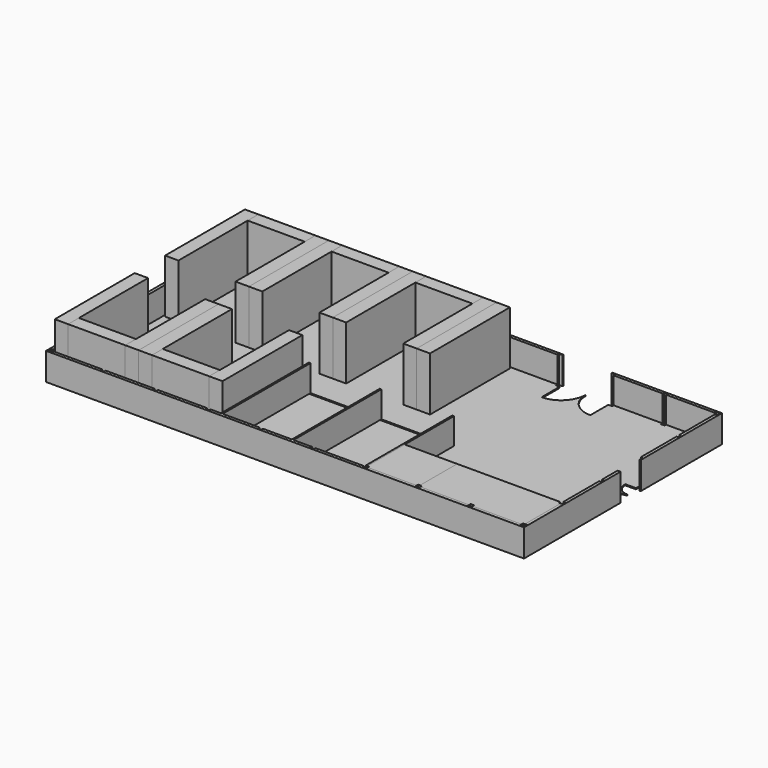
from build123d import *

# Parameters (mm, degrees)
F0_W     = 4500
F0_H     = 1300
F1_DEPTH = 100
F2_DEPTH = 5000
F3_DEPTH = 5000
F4_DEPTH = 5000
F0_W_2   = 150
F0_H_2   = 9850
F0_H_3   = 150
F5_DEPTH = 2500
F6_DEPTH = 2500
F7_DEPTH = 2500
F8_DEPTH = 2500


# Not quite as in the source:
# - a feature names something its author has since deleted; it is built from what else it names


with BuildPart() as f1:
    # F0 (on Top) → F1 (new body)
    with BuildSketch(Plane.XY):
        with BuildLine():
            ThreePointArc((33274.4446, 19781.1111), (31705.4532121104, 20431.0086121104), (31055.5557, 22000))
            ThreePointArc((31055.5557, 22000), (30405.6581878896, 20431.0086121104), (28836.6668, 19781.1111))
            Line((28836.6668, 19781.1111), (28836.6668, 21830))
            Line((28836.6668, 21830), (28496.6668, 21830))
            Line((28496.6668, 21830), (28496.6668, 22000))
            Line((28496.6668, 22000), (24058.889, 22000))
            Line((24058.889, 22000), (24058.889, 21830))
            Line((24058.889, 21830), (24310, 21830))
            Line((24310, 21830), (24310, 12730))
            Line((24310, 12730), (23090, 12730))
            Line((23090, 12730), (21870, 12730))
            Line((21870, 12730), (21870, 20610))
            Line((21870, 20610), (16670, 20610))
            Line((16670, 20610), (16670, 12730))
            Line((16670, 12730), (15450, 12730))
            Line((15450, 12730), (14230, 12730))
            Line((14230, 12730), (14230, 20610))
            Line((14230, 20610), (9030, 20610))
            Line((9030, 20610), (9030, 12730))
            Line((9030, 12730), (7810, 12730))
            Line((7810, 12730), (6590, 12730))
            Line((6590, 12730), (6590, 20610))
            Line((6590, 20610), (1390, 20610))
            Line((1390, 20610), (1390, 12730))
            Line((1390, 12730), (170, 12730))
            Line((170, 12730), (170, 13030))
            Line((170, 13030), (0, 13030))
            Line((0, 13030), (0, 12000))
            Line((0, 12000), (0, 10000))
            Line((0, 10000), (15450, 10000))
            Line((15450, 10000), (15600, 10000))
            Line((15600, 10000), (21908.3334, 10000))
            Line((21908.3334, 10000), (22058.3334, 10000))
            Line((22058.3334, 10000), (28516.6668, 10000))
            Line((28516.6668, 10000), (28666.6668, 10000))
            Line((28666.6668, 10000), (28666.6668, 4400))
            Line((28666.6668, 4400), (33444.4446, 4400))
            Line((33444.4446, 4400), (42830, 4400))
            Line((42830, 4400), (42830, 4570))
            Line((42830, 4570), (43000, 4570))
            Line((43000, 4570), (43000, 8630))
            Line((43000, 8630), (42830, 8630))
            Line((42830, 8630), (42830, 8970))
            Line((42830, 8970), (43000, 8970))
            Line((43000, 8970), (43000, 10730))
            Line((43000, 10730), (41850, 10730))
            ThreePointArc((41850, 10730), (42186.8272016355, 11543.1727983645), (43000, 11880))
            ThreePointArc((43000, 11880), (42186.8272016355, 12216.8272016355), (41850, 13030))
            Line((41850, 13030), (42830, 13030))
            Line((42830, 13030), (42830, 13370))
            Line((42830, 13370), (43000, 13370))
            Line((43000, 13370), (43000, 17430))
            Line((43000, 17430), (42830, 17430))
            Line((42830, 17430), (42830, 17770))
            Line((42830, 17770), (43000, 17770))
            Line((43000, 17770), (43000, 21830))
            Line((43000, 21830), (42830.0002, 21830))
            Line((42830.0002, 21830), (42830.0002, 22000))
            Line((42830.0002, 22000), (38392.2224, 22000))
            Line((38392.2224, 22000), (38392.2224, 21830))
            Line((38392.2224, 21830), (38052.2224, 21830))
            Line((38052.2224, 21830), (38052.2224, 22000))
            Line((38052.2224, 22000), (33614.4446, 22000))
            Line((33614.4446, 22000), (33614.4446, 21830))
            Line((33614.4446, 21830), (33274.4446, 21830))
            Line((33274.4446, 21830), (33274.4446, 19781.1111))
        make_face()
        with Locations((3865.0875091553, 17252.7908325195)):
            Rectangle(F0_W, F0_H, mode=Mode.SUBTRACT)
        with Locations((3865.0875091553, 17252.7908325195)):
            Rectangle(F0_W, F0_H)
        Polygon((15450, 10000), (0, 10000), (0, 8970), (170, 8970), (170, 9270), (1390, 9270), (1390, 1390), (6590, 1390), (6590, 9270), (7810, 9270), (9030, 9270), (9030, 1390), (14230, 1390), (14230, 9270), (15450, 9270), align=None)
        Polygon((33444.4446, 170), (33444.4446, 4400), (28666.6668, 4400), (28666.6668, 170), (28836.6668, 170), (28836.6668, 0), (33274.4446, 0), (33274.4446, 170), align=None)
        Polygon((43000.0001922727, 170), (43000.0000077273, 4230), (42830, 4230), (42830, 4400), (33444.4446, 4400), (33444.4446, 170), (33614.4446, 170), (33614.4446, 0), (38052.2224, 0), (38052.2224, 170), (38392.2224, 170), (38392.2224, 0), (42830.0002, 0), (42830.0002, 170), align=None)
    extrude(amount=F1_DEPTH)

    # F0 (on Top) → F5 (join)
    with BuildSketch(Plane.XY):
        Polygon((15600, 9850), (15600, 10000), (15450, 10000), (15450, 9270), (15450, 170), (15450, 0), (15600, 0), align=None)
        with Locations((21983.3334, 4925)):
            Rectangle(F0_W_2, F0_H_2)
        with Locations((21983.3334, 9925)):
            Rectangle(F0_W_2, F0_H_3)
        Polygon((28666.6668, 170), (28666.6668, 4400), (28666.6668, 10000), (28516.6668, 10000), (28516.6668, 9850), (28516.6668, 4400), (28516.6668, 170), align=None)
    extrude(amount=F5_DEPTH)

    # F0 (on Top) → F6 (join)
    with BuildSketch(Plane.XY):
        Polygon((24058.889, 22000), (28496.6668, 22000), (28496.6668, 22170), (28836.6668, 22170), (28836.6668, 22270), (-270, 22270), (-270, -270), (43270.0002, -270), (43270.0002, 10730), (43000, 10730), (43000, 8970), (43170, 8970), (43170, 8630), (43000, 8630), (43000, 4570), (43170, 4570), (43170, 4230), (43000.0000077273, 4230), (43000.0001922727, 170), (43170.0002, 170), (43170.0002, -170), (42830.0002, -170), (42830.0002, 0), (38392.2224, 0), (38392.2224, -170), (38052.2224, -170), (38052.2224, 0), (33614.4446, 0), (33614.4446, -170), (33274.4446, -170), (33274.4446, 0), (28836.6668, 0), (28836.6668, -170), (28496.6668, -170), (28496.6668, 0), (24058.889, 0), (24058.889, -170), (23718.889, -170), (23718.889, 0), (22058.3334, 0), (21908.3334, 0), (19281.1112, 0), (19281.1112, -170), (18941.1112, -170), (18941.1112, 0), (15600, 0), (15450, 0), (14503.3334, 0), (14503.3334, -170), (14163.3334, -170), (14163.3334, 0), (9725.5556, 0), (9725.5556, -170), (9385.5556, -170), (9385.5556, 0), (4947.7778, 0), (4947.7778, -170), (4607.7778, -170), (4607.7778, 0), (170, 0), (170, -170), (-170, -170), (-170, 170), (0, 170), (0, 4230), (-170, 4230), (-170, 4570), (0, 4570), (0, 8630), (-170, 8630), (-170, 8970), (0, 8970), (0, 10000), (0, 12000), (0, 13030), (-170, 13030), (-170, 13370), (0, 13370), (0, 17430), (-170, 17430), (-170, 17770), (0, 17770), (0, 21830), (-170, 21830), (-170, 22170), (170, 22170), (170, 22000), (4607.7778, 22000), (4607.7778, 22170), (4947.7778, 22170), (4947.7778, 22000), (9385.5556, 22000), (9385.5556, 22170), (9725.5556, 22170), (9725.5556, 22000), (14163.3334, 22000), (14163.3334, 22170), (14503.3334, 22170), (14503.3334, 22000), (18941.1112, 22000), (18941.1112, 22170), (19281.1112, 22170), (19281.1112, 22000), (23718.889, 22000), (23718.889, 22170), (24058.889, 22170), align=None)
        Polygon((33614.4446, 22170), (33614.4446, 22000), (38052.2224, 22000), (38052.2224, 22170), (38392.2224, 22170), (38392.2224, 22000), (42830.0002, 22000), (42830.0002, 22170), (43170.0002, 22170), (43170.0002, 21830), (43000, 21830), (43000, 17770), (43170, 17770), (43170, 17430), (43000, 17430), (43000, 13370), (43170, 13370), (43170, 13030), (43270.0002, 13030), (43270.0002, 22270), (33274.4446, 22270), (33274.4446, 22170), align=None)
    extrude(amount=F6_DEPTH)


with BuildPart() as f1b:
    # F0 (on Top) → F1, piece 2 (new body)
    with BuildSketch(Plane.XY):
        Polygon((28496.6668, 170), (28516.6668, 170), (28516.6668, 4400), (28516.6668, 9850), (22058.3334, 9850), (22058.3334, 0), (23718.889, 0), (23718.889, 170), (24058.889, 170), (24058.889, 0), (28496.6668, 0), align=None)
    extrude(amount=F1_DEPTH)


with BuildPart() as f1c:
    # F0 (on Top) → F1, piece 3 (new body)
    with BuildSketch(Plane.XY):
        Polygon((21908.3334, 0), (21908.3334, 9850), (15600, 9850), (15600, 0), (18941.1112, 0), (18941.1112, 170), (19281.1112, 170), (19281.1112, 0), align=None)
    extrude(amount=F1_DEPTH)


with BuildPart() as f2:
    # F0 (on Top) → F2 (new body)
    with BuildSketch(Plane.XY):
        Polygon((7810, 21830), (6590, 21830), (6590, 20610), (6590, 12730), (7810, 12730), align=None)
    extrude(amount=F2_DEPTH)


with BuildPart() as f2b:
    # F0 (on Top) → F2, piece 2 (new body)
    with BuildSketch(Plane.XY):
        Polygon((1390, 21830), (170, 21830), (170, 17770), (170, 17430), (170, 13370), (170, 13030), (170, 12730), (1390, 12730), (1390, 20610), align=None)
    extrude(amount=F2_DEPTH)


with BuildPart() as f2c:
    # F0 (on Top) → F2, piece 3 (new body)
    with BuildSketch(Plane.XY):
        Polygon((15450, 21830), (14503.3334, 21830), (14230, 21830), (14230, 20610), (14230, 12730), (15450, 12730), align=None)
    extrude(amount=F2_DEPTH)


with BuildPart() as f2d:
    # F0 (on Top) → F2, piece 4 (new body)
    with BuildSketch(Plane.XY):
        Polygon((23090, 12730), (23090, 21830), (21870, 21830), (21870, 20610), (21870, 12730), align=None)
    extrude(amount=F2_DEPTH)


with BuildPart() as f2e:
    # F0 (on Top) → F2, piece 5 (new body)
    with BuildSketch(Plane.XY):
        Polygon((170, 9270), (170, 8970), (170, 8630), (170, 4570), (170, 4230), (170, 170), (1390, 170), (1390, 1390), (1390, 9270), align=None)
    extrude(amount=F2_DEPTH)


with BuildPart() as f2f:
    # F0 (on Top) → F2, piece 6 (new body)
    with BuildSketch(Plane.XY):
        Polygon((6590, 9270), (6590, 1390), (6590, 170), (7810, 170), (7810, 9270), align=None)
    extrude(amount=F2_DEPTH)


with BuildPart() as f2g:
    # F0 (on Top) → F2, piece 7 (new body)
    with BuildSketch(Plane.XY):
        Polygon((15450, 170), (15450, 9270), (14230, 9270), (14230, 1390), (14230, 170), (14503.3334, 170), align=None)
    extrude(amount=F2_DEPTH)


with BuildPart() as f3:
    # F0 (on Top) → F3 (new body)
    with BuildSketch(Plane.XY):
        Polygon((9030, 12730), (9030, 20610), (9030, 21830), (7810, 21830), (7810, 12730), align=None)
    extrude(amount=F3_DEPTH)


with BuildPart() as f3b:
    # F0 (on Top) → F3, piece 2 (new body)
    with BuildSketch(Plane.XY):
        Polygon((16670, 20610), (16670, 21830), (15450, 21830), (15450, 12730), (16670, 12730), align=None)
    extrude(amount=F3_DEPTH)


with BuildPart() as f3c:
    # F0 (on Top) → F3, piece 3 (new body)
    with BuildSketch(Plane.XY):
        Polygon((24310, 21830), (24058.889, 21830), (23718.889, 21830), (23090, 21830), (23090, 12730), (24310, 12730), align=None)
    extrude(amount=F3_DEPTH)


with BuildPart() as f3d:
    # F0 (on Top) → F3, piece 4 (new body)
    with BuildSketch(Plane.XY):
        Polygon((9030, 170), (9030, 1390), (9030, 9270), (7810, 9270), (7810, 170), align=None)
    extrude(amount=F3_DEPTH)


with BuildPart() as f4:
    # F0 (on Top) → F4 (new body)
    with BuildSketch(Plane.XY):
        Polygon((6590, 21830), (4947.7778, 21830), (4607.7778, 21830), (1390, 21830), (1390, 20610), (6590, 20610), align=None)
    extrude(amount=F4_DEPTH)


with BuildPart() as f4b:
    # F0 (on Top) → F4, piece 2 (new body)
    with BuildSketch(Plane.XY):
        Polygon((14230, 21830), (14163.3334, 21830), (9725.5556, 21830), (9385.5556, 21830), (9030, 21830), (9030, 20610), (14230, 20610), align=None)
    extrude(amount=F4_DEPTH)


with BuildPart() as f4c:
    # F0 (on Top) → F4, piece 3 (new body)
    with BuildSketch(Plane.XY):
        Polygon((21870, 21830), (19281.1112, 21830), (18941.1112, 21830), (16670, 21830), (16670, 20610), (21870, 20610), align=None)
    extrude(amount=F4_DEPTH)


with BuildPart() as f4d:
    # F0 (on Top) → F4, piece 4 (new body)
    with BuildSketch(Plane.XY):
        Polygon((6590, 1390), (1390, 1390), (1390, 170), (4607.7778, 170), (4947.7778, 170), (6590, 170), align=None)
    extrude(amount=F4_DEPTH)


with BuildPart() as f4e:
    # F0 (on Top) → F4, piece 5 (new body)
    with BuildSketch(Plane.XY):
        Polygon((14230, 170), (14230, 1390), (9030, 1390), (9030, 170), (9385.5556, 170), (9725.5556, 170), (14163.3334, 170), align=None)
    extrude(amount=F4_DEPTH)


with BuildPart() as f7:
    # F0 (on Top) → F7 (new body)
    with BuildSketch(Plane.XY):
        Polygon((33444.4446, 170), (33444.4446, 4400), (28666.6668, 4400), (28666.6668, 170), (28836.6668, 170), (28836.6668, 0), (33274.4446, 0), (33274.4446, 170), align=None)
    extrude(amount=F7_DEPTH)


with BuildPart() as f8:
    # F0 (on Top) → F8 (new body)
    with BuildSketch(Plane.XY):
        Polygon((43000.0001922727, 170), (43000.0000077273, 4230), (42830, 4230), (42830, 4400), (33444.4446, 4400), (33444.4446, 170), (33614.4446, 170), (33614.4446, 0), (38052.2224, 0), (38052.2224, 170), (38392.2224, 170), (38392.2224, 0), (42830.0002, 0), (42830.0002, 170), align=None)
    extrude(amount=F8_DEPTH)


solid = Compound([f1.part, f1b.part, f1c.part, f2.part, f2b.part, f2c.part, f2d.part, f2e.part, f2f.part, f2g.part, f3.part, f3b.part, f3c.part, f3d.part, f4.part, f4b.part, f4c.part, f4d.part, f4e.part, f7.part, f8.part])
